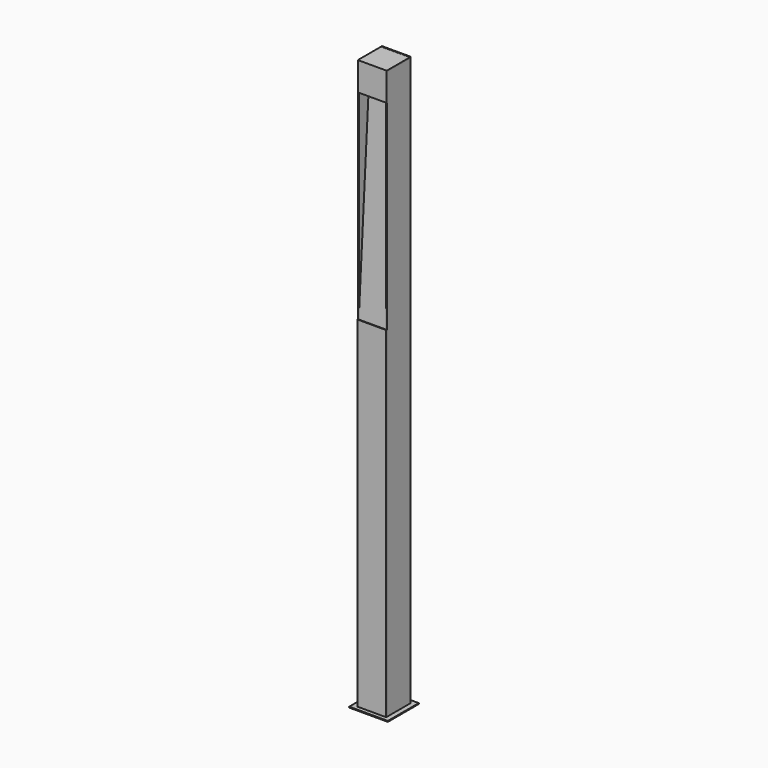
from build123d import *

# Parameters (mm, degrees)
F1_DEPTH  = 3000
F2_W      = 152.4
F2_H      = 152.4
F3_DEPTH  = 4.7625
F4_W      = 151.6622528434
F4_H      = 3006.1117890291
F5_DEPTH  = 4.7625
F6_W      = 152.4
F6_H      = 150
F7_DEPTH  = 1.21
F9_DEPTH  = 71.464
F10_W     = 152.4
F10_H     = 1800
F11_DEPTH = 4.7625
F12_W     = 204
F12_H     = 204
F13_DEPTH = 4.763


# Not quite as in the source:
# - a length typed as a fraction of an inch, garbled in the dataset ("3 / 203.2 mm" for 3/8 in), is restored


with BuildPart() as f1:
    # F0 (on Top) → F1 (new body)
    with BuildSketch(Plane.XY):
        Polygon((-76.2, 76.2), (-76.2, -76.2), (-71.437, -76.2), (-71.437, -2.3815), (71.437, -2.3815), (71.437, -76.2), (76.2, -76.2), (76.2, 76.2), (71.437, 76.2), (71.437, 2.382), (-71.437, 2.382), (-71.437, 76.2), align=None)
    extrude(amount=-F1_DEPTH)

    # F8 (on Right) → F9 (join, symmetric)
    with BuildSketch(Plane.YZ):
        Polygon((-0.7011980658, 4.2686027455), (-1.9099500496, 4.323544912), (-77.5102381694, -1199.9238790681), (-76.3098538914, -1200.0761209319), align=None)
    extrude(amount=F9_DEPTH, both=True)


with BuildPart() as f3:
    # F2 (on face) → F3 (new body)
    with BuildSketch(Plane.XY):
        Rectangle(F2_W, F2_H)
    extrude(amount=F3_DEPTH)


with BuildPart() as f5:
    # F4 (on face) → F5 (new body)
    with BuildSketch(Plane(origin=(0, 76.2, 0), x_dir=(-1, 0, 0), z_dir=(0, 1, 0))):
        with Locations((-0.2847127616, -1497.5008128677)):
            Rectangle(F4_W, F4_H)
    extrude(amount=F5_DEPTH)


with BuildPart() as f7:
    # F6 (on face) → F7 (new body)
    with BuildSketch(Plane.XZ.offset(76.2)):
        with Locations((0, -70.2375)):
            Rectangle(F6_W, F6_H)
    extrude(amount=F7_DEPTH)


with BuildPart() as f11:
    # F10 (on face) → F11 (new body)
    with BuildSketch(Plane.XZ.offset(76.2)):
        with Locations((0, -2100)):
            Rectangle(F10_W, F10_H)
    extrude(amount=F11_DEPTH)


with BuildPart() as f13:
    # F12 (on face) → F13 (new body)
    with BuildSketch(Plane(origin=(0, 0, -3000), x_dir=(1, 0, 0), z_dir=(0, 0, -1))):
        Rectangle(F12_W, F12_H)
    extrude(amount=F13_DEPTH)


solid = Compound([f1.part, f3.part, f5.part, f7.part, f11.part, f13.part])
